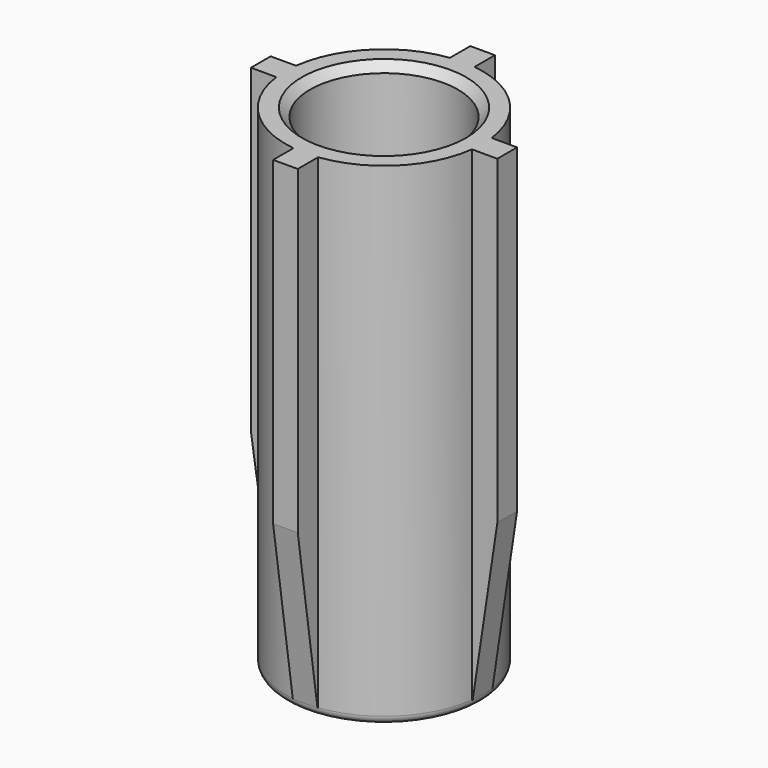
from build123d import *

# Parameters (mm, degrees)
F1_R        = 6
F1_R_2      = 4.5
F2_DEPTH    = 30
F4_W        = 1.5
F4_H        = 2.639524132
F5_DEPTH    = 29.5
F6_COUNT    = 4
F8_R        = 4.5
F8_R_2      = 2.25
F9_DEPTH    = 1.5
F10_SIZE2   = 1.49999
F10_SIZE    = 9.99999
F10_2_SIZE2 = 1.49999
F10_2_SIZE  = 9.99999
F10_3_SIZE2 = 1.49999
F10_3_SIZE  = 9.99999
F10_4_SIZE2 = 1.49999
F10_4_SIZE  = 9.99999
F11_SIZE    = 0.5
F12_R       = 0.49999


# Not quite as in the source:
# - a fillet or chamfer is up to 0.001 mm smaller than in the source, because OpenCascade refuses the exact size


with BuildPart() as f2:
    # F1 (on offset) → F2 (new body)
    with BuildSketch(Plane.XY):
        with Locations((-25, 25)):
            Circle(F1_R)
        with Locations((-25, 25)):
            Circle(F1_R_2, mode=Mode.SUBTRACT)
    extrude(amount=-F2_DEPTH)

    # F4 (on offset) → F5 (join)
    with BuildSketch(Plane.XY):
        with Locations((-25, 31.180237934)):
            Rectangle(F4_W, F4_H)
    extrude(amount=-F5_DEPTH)

    # F6: F2 ×4 about axis
    f6_axis = Axis((-25, 25, 0), (0, 0, 1))


with BuildPart() as f2_1:
    add(f2.part)
    for i in range(1, F6_COUNT):
        add(f2.part.rotate(f6_axis, i * 360 / F6_COUNT))

    # F8 (on offset) → F9 (join)
    with BuildSketch(Plane.XY.offset(-30)):
        with Locations((-25, 25)):
            Circle(F8_R)
        with Locations((-25, 25)):
            Circle(F8_R_2, mode=Mode.SUBTRACT)
    extrude(amount=F9_DEPTH)

    # F10 (size 10 and 1.5 in the source; OpenCascade refuses exactly that, so slightly less here)
    f10_edges = [f2_1.edges().sort_by_distance(p)[0] for p in [
        (-25, 17.5, -29.5),
    ]]
    f10_side = f2_1.faces().sort_by_distance((-25, 17.5, -14.75))[0]
    chamfer(f10_edges, length=F10_SIZE, length2=F10_SIZE2, reference=f10_side)

    # F10#2 (size 10 and 1.5 in the source; OpenCascade refuses exactly that, so slightly less here)
    f10_2_edges = [f2_1.edges().sort_by_distance(p)[0] for p in [
        (-17.5, 25, -29.5),
    ]]
    f10_2_side = f2_1.faces().sort_by_distance((-17.5, 25, -14.75))[0]
    chamfer(f10_2_edges, length=F10_2_SIZE, length2=F10_2_SIZE2, reference=f10_2_side)

    # F10#3 (size 10 and 1.5 in the source; OpenCascade refuses exactly that, so slightly less here)
    f10_3_edges = [f2_1.edges().sort_by_distance(p)[0] for p in [
        (-25, 32.5, -29.5),
    ]]
    f10_3_side = f2_1.faces().sort_by_distance((-25, 32.5, -14.75))[0]
    chamfer(f10_3_edges, length=F10_3_SIZE, length2=F10_3_SIZE2, reference=f10_3_side)

    # F10#4 (size 10 and 1.5 in the source; OpenCascade refuses exactly that, so slightly less here)
    f10_4_edges = [f2_1.edges().sort_by_distance(p)[0] for p in [
        (-32.5, 25, -29.5),
    ]]
    f10_4_side = f2_1.faces().sort_by_distance((-32.5, 25, -14.75))[0]
    chamfer(f10_4_edges, length=F10_4_SIZE, length2=F10_4_SIZE2, reference=f10_4_side)

    # F11
    f11_edges = [f2_1.edges().sort_by_distance(p)[0] for p in [
        (-29.5, 25, 0),
        (-27.25, 25, -28.5),
    ]]
    chamfer(f11_edges, length=F11_SIZE)

    # F12 (radius 0.5 in the source; OpenCascade refuses exactly that, so slightly less here)
    f12_edges = [f2_1.edges().sort_by_distance(p)[0] for p in [
        (-31, 25, -30),
    ]]
    fillet(f12_edges, radius=F12_R)


solid = f2_1.part
